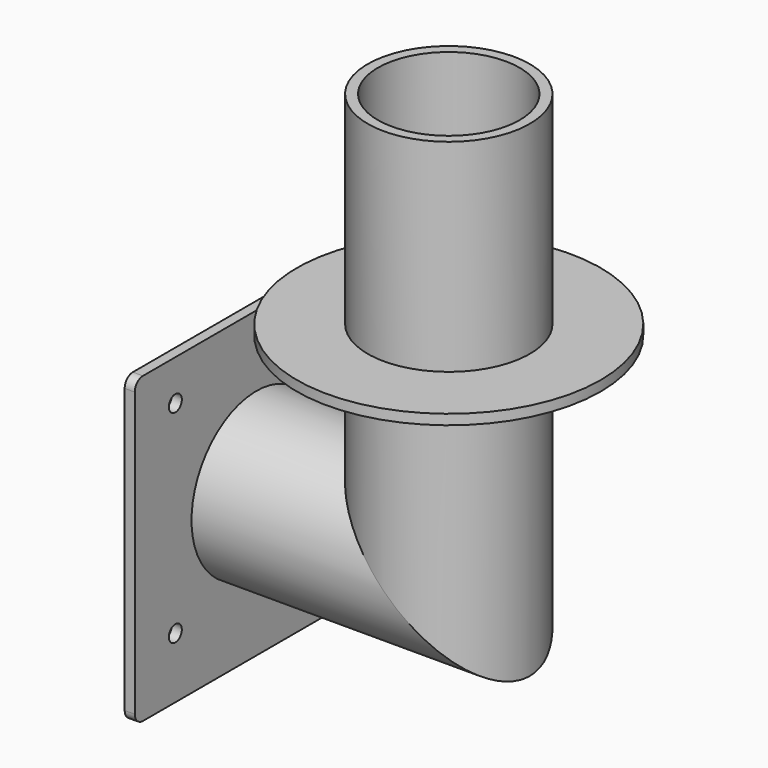
from build123d import *

# Parameters (mm, degrees)
F0_R     = 40
F0_R_2   = 34.9999991059
F5_R     = 75
F5_R_2   = 40
F6_DEPTH = 5
F2_R     = 4
F7_DEPTH = 5


with BuildPart() as f3:
    # F3: sweep along a path in F1
    with BuildLine(Plane.XZ) as f3_path:
        Line((0, 0), (100, 0))
        Line((100, 0), (100, 200))
    # F0 (on Right) → F3 (sweep)
    with BuildSketch(Plane.YZ):
        Circle(F0_R)
        Circle(F0_R_2, mode=Mode.SUBTRACT)
    sweep(path=f3_path.line, transition=Transition.RIGHT)

    # F5 (on face) → F6 (join)
    with BuildSketch(Plane.XY.offset(100)):
        with Locations((100, 0)):
            Circle(F5_R)
        with Locations((100, 0)):
            Circle(F5_R_2, mode=Mode.SUBTRACT)
    extrude(amount=-F6_DEPTH)

    # F2 (on Right) → F7 (join)
    with BuildSketch(Plane.YZ):
        with BuildLine():
            Line((-70, -75), (70, -75))
            ThreePointArc((70, -75), (73.5355339059, -73.5355339059), (75, -70))
            Line((75, -70), (75, 70))
            ThreePointArc((75, 70), (73.5355339059, 73.5355339059), (70, 75))
            Line((70, 75), (-70, 75))
            ThreePointArc((-70, 75), (-73.5355339059, 73.5355339059), (-75, 70))
            Line((-75, 70), (-75, -70))
            ThreePointArc((-75, -70), (-73.5355339059, -73.5355339059), (-70, -75))
        make_face()
        with Locations((-50, -45)):
            Circle(F2_R, mode=Mode.SUBTRACT)
        with Locations((50, -45)):
            Circle(F2_R, mode=Mode.SUBTRACT)
        with Locations((-50, 55)):
            Circle(F2_R, mode=Mode.SUBTRACT)
        with Locations((50, 55)):
            Circle(F2_R, mode=Mode.SUBTRACT)
    extrude(amount=F7_DEPTH)


solid = f3.part
